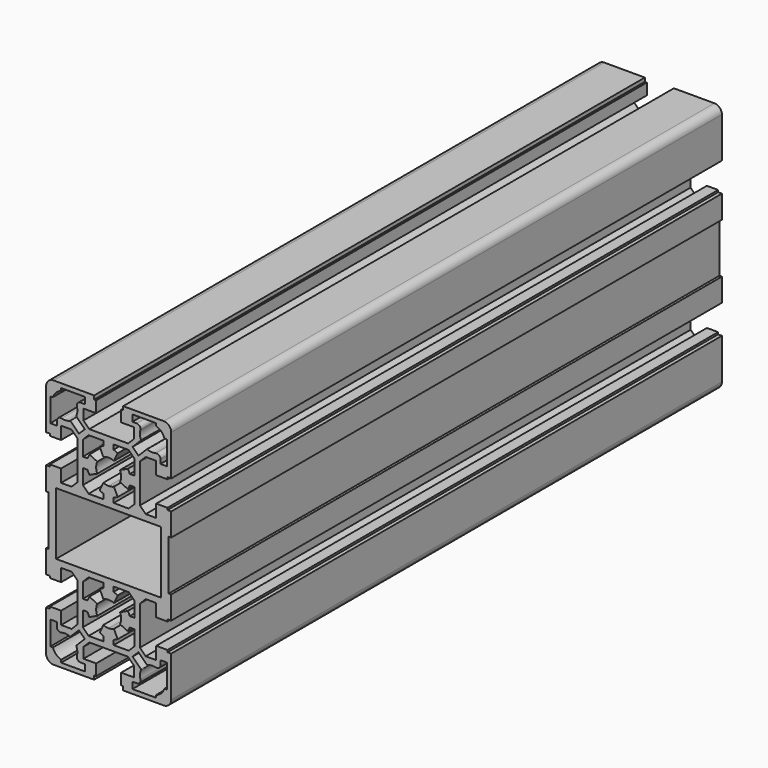
from build123d import *

# Parameters (mm, degrees)
F3_DEPTH = 275


# Not quite as in the source:
# - ends of sketch curves that miss each other by under 0.0002 mm in the source are joined


with BuildPart() as f3:
    # F2 (on Front) → F3 (new body)
    with BuildSketch(Plane.XZ):
        with BuildLine():
            Line((21.000169, 12.449667), (21.000169, -0.000333))
            Line((21.000169, -0.000333), (24.000169, -0.000333))
            Line((24.000169, -0.000333), (24.000169, 9.999667))
            Line((24.000169, 9.999667), (25.000169, 9.999667))
            Line((25.000169, 9.999667), (25.000169, 19.199667))
            Line((25.000169, 19.199667), (23.500169, 19.199667))
            Line((23.500169, 19.199667), (23.500169, 19.999667))
            Line((23.500169, 19.999667), (19.000169, 19.999667))
            Line((19.000169, 19.999667), (19.000169, 14.949667))
            Line((19.000169, 14.949667), (14.800169, 14.949667))
            Line((14.800169, 14.949667), (12.500169, 17.249667))
            Line((12.500169, 17.249667), (12.500169, 32.749667))
            Line((12.500169, 32.749667), (14.800169, 35.049667))
            Line((14.800169, 35.049667), (19.000169, 35.049667))
            Line((19.000169, 35.049667), (19.000169, 29.999667))
            Line((19.000169, 29.999667), (23.500169, 29.999667))
            Line((23.500169, 29.999667), (23.500169, 30.799667))
            Line((23.500169, 30.799667), (25.000169, 30.799667))
            Line((25.000169, 30.799667), (25.000169, 46.999667))
            ThreePointArc((25.000169, 46.999667), (24.1214893436, 49.1209873436), (22.000169, 49.999667))
            Line((22.000169, 49.999667), (5.800169, 49.999667))
            Line((5.800169, 49.999667), (5.800169, 48.499667))
            Line((5.800169, 48.499667), (5.000169, 48.499667))
            Line((5.000169, 48.499667), (5.000169, 43.999667))
            Line((5.000169, 43.999667), (10.050169, 43.999667))
            Line((10.050169, 43.999667), (10.050169, 39.799667))
            Line((10.050169, 39.799667), (7.750169, 37.499667))
            Line((7.750169, 37.499667), (0.000169, 37.499667))
            Line((0.000169, 37.499667), (0.000169, 29.999667))
            ThreePointArc((0.000169, 29.999667), (1.0823669197, 29.8811470688), (2.1132600303, 29.531206065))
            Line((2.11326, 29.531206), (3.592424, 32.703283))
            Line((3.592424, 32.703283), (2.000169, 33.445764))
            Line((2.000169, 33.445764), (2.000169, 35.299667))
            Line((2.000169, 35.299667), (8.012449, 35.299667))
            Line((8.012449, 35.299667), (10.300169, 33.011947))
            Line((10.300169, 33.011947), (10.300169, 26.999667))
            Line((10.300169, 26.999667), (8.446266, 26.999667))
            Line((8.446266, 26.999667), (7.703785, 28.591922))
            Line((7.703785, 28.591922), (4.531708, 27.112758))
            ThreePointArc((4.531708065, 27.1127580303), (5.000169, 24.999667), (4.531708065, 22.8865759697))
            Line((4.531708, 22.886576), (7.703785, 21.407412))
            Line((7.703785, 21.407412), (8.446266, 22.999667))
            Line((8.446266, 22.999667), (10.300169, 22.999667))
            Line((10.300169, 22.999667), (10.300169, 16.987387))
            Line((10.300169, 16.987387), (8.012449, 14.699667))
            Line((8.012449, 14.699667), (2.000169, 14.699667))
            Line((2.000169, 14.699667), (2.000169, 16.55357))
            Line((2.000169, 16.55357), (3.592424, 17.296051))
            Line((3.592424, 17.296051), (2.11326, 20.468128))
            ThreePointArc((2.1132600303, 20.468127935), (1.0823669197, 20.1181869312), (0.000169, 19.999667))
            Line((0.000169, 19.999667), (0.000169, 12.449667))
            Line((0.000169, 12.449667), (21.000169, 12.449667))
        make_face()
        with BuildLine():
            Line((20.700169, 34.499667), (20.700169, 36.225912))
            ThreePointArc((20.700169, 36.225912), (20.1116343558, 37.41722678), (18.8078611265, 37.6737015332))
            ThreePointArc((18.8078611265, 37.6737015332), (17.1448966414, 37.5123048163), (15.5216018999, 37.9077967677))
            ThreePointArc((15.5216018999, 37.9077967677), (15.3464434299, 37.9269271737), (15.1907559656, 37.8444170344))
            Line((15.1907559656, 37.8444170344), (11.884862, 34.538523))
            Line((11.884862, 34.538523), (9.539025, 36.88436))
            Line((9.539025, 36.88436), (12.844919, 40.190254))
            ThreePointArc((12.844919, 40.190254), (12.9274291737, 40.3459414299), (12.9082991899, 40.5211000818))
            ThreePointArc((12.9082991899, 40.5211000818), (12.5128068163, 42.1443946414), (12.6742036668, 43.8073590903))
            ThreePointArc((12.6742036668, 43.8073590903), (12.41772878, 45.1111323558), (11.226414, 45.699667))
            Line((11.226414, 45.699667), (9.500169, 45.699667))
            Line((9.500169, 45.699667), (9.500169, 48.299667))
            Line((9.500169, 48.299667), (19.000169, 48.299667))
            Line((19.000169, 48.299667), (19.000169, 47.269363))
            ThreePointArc((19.000169, 47.269363), (21.0357029059, 46.0352009059), (22.2698650064, 43.999667002))
            Line((22.2698650064, 43.999667002), (23.300169, 43.999667))
            Line((23.300169, 43.999667), (23.300169, 34.499667))
            Line((23.300169, 34.499667), (20.700169, 34.499667))
        make_face(mode=Mode.SUBTRACT)
        with BuildLine():
            Line((-23.999831, -0.000333), (-20.999831, -0.000333))
            Line((-20.999831, -0.000333), (-20.999831, 12.449667))
            Line((-20.999831, 12.449667), (0.000169, 12.449667))
            Line((0.000169, 12.449667), (0.000169, 19.999667))
            ThreePointArc((0.000169, 19.999667), (-1.0820289197, 20.1181869312), (-2.1129220303, 20.468127935))
            Line((-2.112922, 20.468128), (-3.592086, 17.296051))
            Line((-3.592086, 17.296051), (-1.999831, 16.55357))
            Line((-1.999831, 16.55357), (-1.999831, 14.699667))
            Line((-1.999831, 14.699667), (-8.012111, 14.699667))
            Line((-8.012111, 14.699667), (-10.299831, 16.987387))
            Line((-10.299831, 16.987387), (-10.299831, 22.999667))
            Line((-10.299831, 22.999667), (-8.445928, 22.999667))
            Line((-8.445928, 22.999667), (-7.703447, 21.407412))
            Line((-7.703447, 21.407412), (-4.53137, 22.886576))
            ThreePointArc((-4.531370065, 22.8865759697), (-4.999831, 24.999667), (-4.531370065, 27.1127580303))
            Line((-4.53137, 27.112758), (-7.703447, 28.591922))
            Line((-7.703447, 28.591922), (-8.445928, 26.999667))
            Line((-8.445928, 26.999667), (-10.299831, 26.999667))
            Line((-10.299831, 26.999667), (-10.299831, 33.011947))
            Line((-10.299831, 33.011947), (-8.012111, 35.299667))
            Line((-8.012111, 35.299667), (-1.999831, 35.299667))
            Line((-1.999831, 35.299667), (-1.999831, 33.445764))
            Line((-1.999831, 33.445764), (-3.592086, 32.703283))
            Line((-3.592086, 32.703283), (-2.112922, 29.531206))
            ThreePointArc((-2.1129220303, 29.531206065), (-1.0820289197, 29.8811470688), (0.000169, 29.999667))
            Line((0.000169, 29.999667), (0.000169, 37.499667))
            Line((0.000169, 37.499667), (-7.749831, 37.499667))
            Line((-7.749831, 37.499667), (-10.049831, 39.799667))
            Line((-10.049831, 39.799667), (-10.049831, 43.999667))
            Line((-10.049831, 43.999667), (-4.999831, 43.999667))
            Line((-4.999831, 43.999667), (-4.999831, 48.499667))
            Line((-4.999831, 48.499667), (-5.799831, 48.499667))
            Line((-5.799831, 48.499667), (-5.799831, 49.999667))
            Line((-5.799831, 49.999667), (-21.999831, 49.999667))
            ThreePointArc((-21.999831, 49.999667), (-24.1211513436, 49.1209873436), (-24.999831, 46.999667))
            Line((-24.999831, 46.999667), (-24.999831, 30.799667))
            Line((-24.999831, 30.799667), (-23.499831, 30.799667))
            Line((-23.499831, 30.799667), (-23.499831, 29.999667))
            Line((-23.499831, 29.999667), (-18.999831, 29.999667))
            Line((-18.999831, 29.999667), (-18.999831, 35.049667))
            Line((-18.999831, 35.049667), (-14.799831, 35.049667))
            Line((-14.799831, 35.049667), (-12.499831, 32.749667))
            Line((-12.499831, 32.749667), (-12.499831, 17.249667))
            Line((-12.499831, 17.249667), (-14.799831, 14.949667))
            Line((-14.799831, 14.949667), (-18.999831, 14.949667))
            Line((-18.999831, 14.949667), (-18.999831, 19.999667))
            Line((-18.999831, 19.999667), (-23.499831, 19.999667))
            Line((-23.499831, 19.999667), (-23.499831, 19.199667))
            Line((-23.499831, 19.199667), (-24.999831, 19.199667))
            Line((-24.999831, 19.199667), (-24.999831, 9.999667))
            Line((-24.999831, 9.999667), (-23.999831, 9.999667))
            Line((-23.999831, 9.999667), (-23.999831, -0.000333))
        make_face()
        with BuildLine():
            ThreePointArc((-15.5212638999, 37.9077967677), (-17.1445586414, 37.5123048163), (-18.8075230903, 37.6737016668))
            ThreePointArc((-18.8075230903, 37.6737016668), (-20.1112963558, 37.41722678), (-20.699831, 36.225912))
            Line((-20.699831, 36.225912), (-20.699831, 34.499667))
            Line((-20.699831, 34.499667), (-23.299831, 34.499667))
            Line((-23.299831, 34.499667), (-23.299831, 43.999667))
            Line((-23.299831, 43.999667), (-22.269527, 43.999667))
            ThreePointArc((-22.269527, 43.999667), (-21.0353649059, 46.0352009059), (-18.999831002, 47.2693630064))
            Line((-18.999831002, 47.2693630064), (-18.999831, 48.299667))
            Line((-18.999831, 48.299667), (-9.499831, 48.299667))
            Line((-9.499831, 48.299667), (-9.499831, 45.699667))
            Line((-9.499831, 45.699667), (-11.226076, 45.699667))
            ThreePointArc((-11.226076, 45.699667), (-12.41739078, 45.1111323558), (-12.6738655332, 43.8073591265))
            ThreePointArc((-12.6738655332, 43.8073591265), (-12.5124688163, 42.1443946414), (-12.9079607677, 40.5210998999))
            ThreePointArc((-12.9079607677, 40.5210998999), (-12.9270911737, 40.3459414299), (-12.8445810344, 40.1902539656))
            Line((-12.8445810344, 40.1902539656), (-9.538687, 36.88436))
            Line((-9.538687, 36.88436), (-11.884524, 34.538523))
            Line((-11.884524, 34.538523), (-15.190418, 37.844417))
            ThreePointArc((-15.190418, 37.844417), (-15.3461054299, 37.9269271737), (-15.5212638999, 37.9077967677))
        make_face(mode=Mode.SUBTRACT)
        with BuildLine():
            Line((5.800169, -50.000333), (22.000169, -50.000333))
            ThreePointArc((22.000169, -50.000333), (24.1214893436, -49.1216533436), (25.000169, -47.000333))
            Line((25.000169, -47.000333), (25.000169, -30.800333))
            Line((25.000169, -30.800333), (23.500169, -30.800333))
            Line((23.500169, -30.800333), (23.500169, -30.000333))
            Line((23.500169, -30.000333), (19.000169, -30.000333))
            Line((19.000169, -30.000333), (19.000169, -35.050333))
            Line((19.000169, -35.050333), (14.800169, -35.050333))
            Line((14.800169, -35.050333), (12.500169, -32.750333))
            Line((12.500169, -32.750333), (12.500169, -17.250333))
            Line((12.500169, -17.250333), (14.800169, -14.950333))
            Line((14.800169, -14.950333), (19.000169, -14.950333))
            Line((19.000169, -14.950333), (19.000169, -20.000333))
            Line((19.000169, -20.000333), (23.500169, -20.000333))
            Line((23.500169, -20.000333), (23.500169, -19.200333))
            Line((23.500169, -19.200333), (25.000169, -19.200333))
            Line((25.000169, -19.200333), (25.000169, -10.000333))
            Line((25.000169, -10.000333), (24.000169, -10.000333))
            Line((24.000169, -10.000333), (24.000169, -0.000333))
            Line((24.000169, -0.000333), (21.000169, -0.000333))
            Line((21.000169, -0.000333), (21.000169, -12.450333))
            Line((21.000169, -12.450333), (0.000169, -12.450333))
            Line((0.000169, -12.450333), (0.000169, -20.000333))
            ThreePointArc((0.000169, -20.000333), (1.0823669197, -20.1188529312), (2.1132600303, -20.468793935))
            Line((2.11326, -20.468794), (3.592424, -17.296717))
            Line((3.592424, -17.296717), (2.000169, -16.554236))
            Line((2.000169, -16.554236), (2.000169, -14.700333))
            Line((2.000169, -14.700333), (8.012449, -14.700333))
            Line((8.012449, -14.700333), (10.300169, -16.988053))
            Line((10.300169, -16.988053), (10.300169, -23.000333))
            Line((10.300169, -23.000333), (8.446266, -23.000333))
            Line((8.446266, -23.000333), (7.703785, -21.408078))
            Line((7.703785, -21.408078), (4.531708, -22.887242))
            ThreePointArc((4.531708065, -22.8872419697), (5.000169, -25.000333), (4.531708065, -27.1134240303))
            Line((4.531708, -27.113424), (7.703785, -28.592588))
            Line((7.703785, -28.592588), (8.446266, -27.000333))
            Line((8.446266, -27.000333), (10.300169, -27.000333))
            Line((10.300169, -27.000333), (10.300169, -33.012613))
            Line((10.300169, -33.012613), (8.012449, -35.300333))
            Line((8.012449, -35.300333), (2.000169, -35.300333))
            Line((2.000169, -35.300333), (2.000169, -33.44643))
            Line((2.000169, -33.44643), (3.592424, -32.703949))
            Line((3.592424, -32.703949), (2.11326, -29.531872))
            ThreePointArc((2.1132600303, -29.531872065), (1.0823669197, -29.8818130688), (0.000169, -30.000333))
            Line((0.000169, -30.000333), (0.000169, -37.500333))
            Line((0.000169, -37.500333), (7.750169, -37.500333))
            Line((7.750169, -37.500333), (10.050169, -39.800333))
            Line((10.050169, -39.800333), (10.050169, -44.000333))
            Line((10.050169, -44.000333), (5.000169, -44.000333))
            Line((5.000169, -44.000333), (5.000169, -48.500333))
            Line((5.000169, -48.500333), (5.800169, -48.500333))
            Line((5.800169, -48.500333), (5.800169, -50.000333))
        make_face()
        with BuildLine():
            ThreePointArc((12.6742036668, -43.8080250903), (12.5128068163, -42.1450606414), (12.9082987677, -40.5217658999))
            ThreePointArc((12.9082987677, -40.5217658999), (12.9274291737, -40.3466074299), (12.8449190344, -40.1909199656))
            Line((12.8449190344, -40.1909199656), (9.539025, -36.885026))
            Line((9.539025, -36.885026), (11.884862, -34.539189))
            Line((11.884862, -34.539189), (15.190756, -37.845083))
            ThreePointArc((15.190756, -37.845083), (15.3464434299, -37.9275931737), (15.5216020818, -37.9084631899))
            ThreePointArc((15.5216020818, -37.9084631899), (17.1448966414, -37.5129708163), (18.8078610903, -37.6743676668))
            ThreePointArc((18.8078610903, -37.6743676668), (20.1116343558, -37.41789278), (20.700169, -36.226578))
            Line((20.700169, -36.226578), (20.700169, -34.500333))
            Line((20.700169, -34.500333), (23.300169, -34.500333))
            Line((23.300169, -34.500333), (23.300169, -44.000333))
            Line((23.300169, -44.000333), (22.269865, -44.000333))
            ThreePointArc((22.269865, -44.000333), (21.0357029059, -46.0358669059), (19.000169002, -47.2700290064))
            Line((19.000169002, -47.2700290064), (19.000169, -48.300333))
            Line((19.000169, -48.300333), (9.500169, -48.300333))
            Line((9.500169, -48.300333), (9.500169, -45.700333))
            Line((9.500169, -45.700333), (11.226414, -45.700333))
            ThreePointArc((11.226414, -45.700333), (12.41772878, -45.1117983558), (12.6742036668, -43.8080250903))
        make_face(mode=Mode.SUBTRACT)
        with BuildLine():
            Line((-7.749831, -37.500333), (0.000169, -37.500333))
            Line((0.000169, -37.500333), (0.000169, -30.000333))
            ThreePointArc((0.000169, -30.000333), (-1.0820289197, -29.8818130688), (-2.1129220303, -29.531872065))
            Line((-2.112922, -29.531872), (-3.592086, -32.703949))
            Line((-3.592086, -32.703949), (-1.999831, -33.44643))
            Line((-1.999831, -33.44643), (-1.999831, -35.300333))
            Line((-1.999831, -35.300333), (-8.012111, -35.300333))
            Line((-8.012111, -35.300333), (-10.299831, -33.012613))
            Line((-10.299831, -33.012613), (-10.299831, -27.000333))
            Line((-10.299831, -27.000333), (-8.445928, -27.000333))
            Line((-8.445928, -27.000333), (-7.703447, -28.592588))
            Line((-7.703447, -28.592588), (-4.53137, -27.113424))
            ThreePointArc((-4.531370065, -27.1134240303), (-4.999831, -25.000333), (-4.531370065, -22.8872419697))
            Line((-4.53137, -22.887242), (-7.703447, -21.408078))
            Line((-7.703447, -21.408078), (-8.445928, -23.000333))
            Line((-8.445928, -23.000333), (-10.299831, -23.000333))
            Line((-10.299831, -23.000333), (-10.299831, -16.988053))
            Line((-10.299831, -16.988053), (-8.012111, -14.700333))
            Line((-8.012111, -14.700333), (-1.999831, -14.700333))
            Line((-1.999831, -14.700333), (-1.999831, -16.554236))
            Line((-1.999831, -16.554236), (-3.592086, -17.296717))
            Line((-3.592086, -17.296717), (-2.112922, -20.468794))
            ThreePointArc((-2.1129220303, -20.468793935), (-1.0820289197, -20.1188529312), (0.000169, -20.000333))
            Line((0.000169, -20.000333), (0.000169, -12.450333))
            Line((0.000169, -12.450333), (-20.999831, -12.450333))
            Line((-20.999831, -12.450333), (-20.999831, -0.000333))
            Line((-20.999831, -0.000333), (-23.999831, -0.000333))
            Line((-23.999831, -0.000333), (-23.999831, -10.000333))
            Line((-23.999831, -10.000333), (-24.999831, -10.000333))
            Line((-24.999831, -10.000333), (-24.999831, -19.200333))
            Line((-24.999831, -19.200333), (-23.499831, -19.200333))
            Line((-23.499831, -19.200333), (-23.499831, -20.000333))
            Line((-23.499831, -20.000333), (-18.999831, -20.000333))
            Line((-18.999831, -20.000333), (-18.999831, -14.950333))
            Line((-18.999831, -14.950333), (-14.799831, -14.950333))
            Line((-14.799831, -14.950333), (-12.499831, -17.250333))
            Line((-12.499831, -17.250333), (-12.499831, -32.750333))
            Line((-12.499831, -32.750333), (-14.799831, -35.050333))
            Line((-14.799831, -35.050333), (-18.999831, -35.050333))
            Line((-18.999831, -35.050333), (-18.999831, -30.000333))
            Line((-18.999831, -30.000333), (-23.499831, -30.000333))
            Line((-23.499831, -30.000333), (-23.499831, -30.800333))
            Line((-23.499831, -30.800333), (-24.999831, -30.800333))
            Line((-24.999831, -30.800333), (-24.999831, -47.000333))
            ThreePointArc((-24.999831, -47.000333), (-24.1211513436, -49.1216533436), (-21.999831, -50.000333))
            Line((-21.999831, -50.000333), (-5.799831, -50.000333))
            Line((-5.799831, -50.000333), (-5.799831, -48.500333))
            Line((-5.799831, -48.500333), (-4.999831, -48.500333))
            Line((-4.999831, -48.500333), (-4.999831, -44.000333))
            Line((-4.999831, -44.000333), (-10.049831, -44.000333))
            Line((-10.049831, -44.000333), (-10.049831, -39.800333))
            Line((-10.049831, -39.800333), (-7.749831, -37.500333))
        make_face()
        with BuildLine():
            ThreePointArc((-12.9079607677, -40.5217658999), (-12.5124688163, -42.1450606414), (-12.6738656668, -43.8080250903))
            ThreePointArc((-12.6738656668, -43.8080250903), (-12.41739078, -45.1117983558), (-11.226076, -45.700333))
            Line((-11.226076, -45.700333), (-9.499831, -45.700333))
            Line((-9.499831, -45.700333), (-9.499831, -48.300333))
            Line((-9.499831, -48.300333), (-18.999831, -48.300333))
            Line((-18.999831, -48.300333), (-18.999831, -47.270029))
            ThreePointArc((-18.999831, -47.270029), (-21.0353649059, -46.0358669059), (-22.2695270064, -44.000333002))
            Line((-22.2695270064, -44.000333002), (-23.299831, -44.000333))
            Line((-23.299831, -44.000333), (-23.299831, -34.500333))
            Line((-23.299831, -34.500333), (-20.699831, -34.500333))
            Line((-20.699831, -34.500333), (-20.699831, -36.226578))
            ThreePointArc((-20.699831, -36.226578), (-20.1112963558, -37.41789278), (-18.8075231265, -37.6743675332))
            ThreePointArc((-18.8075231265, -37.6743675332), (-17.1445586414, -37.5129708163), (-15.5212638999, -37.9084627677))
            ThreePointArc((-15.5212638999, -37.9084627677), (-15.3461054299, -37.9275931737), (-15.1904179656, -37.8450830344))
            Line((-15.1904179656, -37.8450830344), (-11.884524, -34.539189))
            Line((-11.884524, -34.539189), (-9.538687, -36.885026))
            Line((-9.538687, -36.885026), (-12.844581, -40.19092))
            ThreePointArc((-12.844581, -40.19092), (-12.9270911737, -40.3466074299), (-12.9079607677, -40.5217658999))
        make_face(mode=Mode.SUBTRACT)
    extrude(amount=-F3_DEPTH)


solid = f3.part
